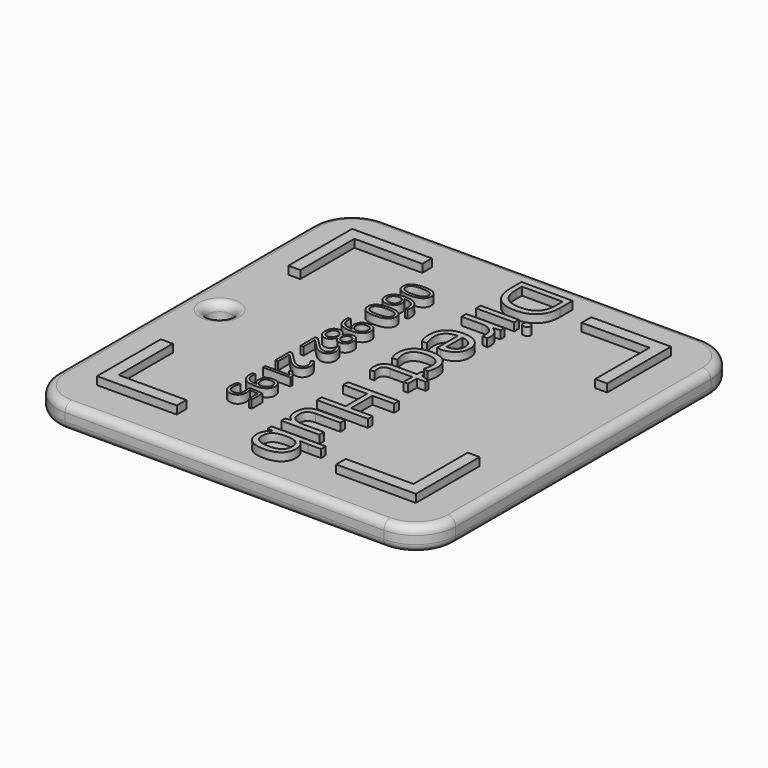
from build123d import *

# Parameters (mm, degrees)
F1_W          = 50
F1_H          = 50
F2_DEPTH      = 3
F4_D          = 3
F5_R          = 1
F6_R          = 1
F7_T1_DEPTH   = 3
F7_T4_ANGLE   = 90
F7_T6_ANGLE   = 90
F7_T8_ANGLE   = 90
F7_T10_ANGLE  = 90
F7_T12_ANGLE  = 90
F7_T14_ANGLE  = 90
F7_T16_ANGLE  = 90
F7_T18_ANGLE  = 90
F8_TEXT_SIZE  = 8.9550794579
F9_DEPTH      = 1
F10_TEXT_SIZE = 4.8044441108
F11_DEPTH     = 1
F13_DEPTH     = 1
F14_DEPTH     = 1


# Not quite as in the source:
# - a fillet or chamfer that OpenCascade refuses, or shapes differently, is made with other operations: its cross-section is extruded or revolved along the edge and cut away or added
# - Text() gives the source's letters only with a copy of the font that has no kerning and outlines rounded to 1/6400 em; it was checked with that copy


with BuildPart() as f2:
    # F1 (on face) → F2 (new body)
    with BuildSketch(Plane.XY):
        Rectangle(F1_W, F1_H)
    extrude(amount=F2_DEPTH)

    # F4 (through all)
    with Locations(Plane.XY.offset(3)):
        with Locations((-20.6191185862, 0)):
            Hole(F4_D / 2)

    # F5
    f5_edges = [f2.edges().sort_by_distance(p)[0] for p in [
        (-25, 0, 3),
        (0, 25, 3),
        (0, -25, 3),
        (25, 0, 3),
        (-22.119119, 0, 3),
    ]]
    fillet(f5_edges, radius=F5_R)

    # F6
    f6_edges = [f2.edges().sort_by_distance(p)[0] for p in [
        (-25, 0, 0),
        (0, 25, 0),
        (0, -25, 0),
        (25, 0, 0),
        (-22.119119, 0, 0),
    ]]
    fillet(f6_edges, radius=F6_R)

    # F7: fillet of radius 5 on 4 edges, made by hand

    # F7_s2 → F7_t1 (cut)
    with BuildSketch(Plane.XY):
        with BuildLine():
            ThreePointArc((-25, 20), (-23.5355339059, 23.5355339059), (-20, 25))
            Line((-20, 25), (-25, 25))
            Line((-25, 25), (-25, 20))
        make_face()
        with BuildLine():
            ThreePointArc((-25, -20), (-23.5355339059, -23.5355339059), (-20, -25))
            Line((-20, -25), (-25, -25))
            Line((-25, -25), (-25, -20))
        make_face()
        with BuildLine():
            ThreePointArc((20, 25), (23.5355339059, 23.5355339059), (25, 20))
            Line((25, 20), (25, 25))
            Line((25, 25), (20, 25))
        make_face()
        with BuildLine():
            ThreePointArc((20, -25), (23.5355339059, -23.5355339059), (25, -20))
            Line((25, -20), (25, -25))
            Line((25, -25), (20, -25))
        make_face()
    extrude(amount=F7_T1_DEPTH, mode=Mode.SUBTRACT)

    # F7_s3 → F7_t4 (revolve, cut)
    with BuildSketch(Plane.XZ.offset(20)):
        with BuildLine():
            ThreePointArc((24, 0), (24.7071067812, 0.2928932188), (25, 1))
            Line((25, 1), (25, 0))
            Line((25, 0), (24, 0))
        make_face()
    revolve(axis=Axis((20, -20, 0), (0, 0, -1)), revolution_arc=F7_T4_ANGLE, mode=Mode.SUBTRACT)

    # F7_s5 → F7_t6 (revolve, cut)
    with BuildSketch(Plane.YZ.offset(20)):
        with BuildLine():
            ThreePointArc((-24, 3), (-24.7071067812, 2.7071067812), (-25, 2))
            Line((-25, 2), (-25, 3))
            Line((-25, 3), (-24, 3))
        make_face()
    revolve(axis=Axis((20, -20, 3), (0, 0, 1)), revolution_arc=F7_T6_ANGLE, mode=Mode.SUBTRACT)

    # F7_s7 → F7_t8 (revolve, cut)
    with BuildSketch(Plane.YZ.offset(20)):
        with BuildLine():
            ThreePointArc((24, 0), (24.7071067812, 0.2928932188), (25, 1))
            Line((25, 1), (25, 0))
            Line((25, 0), (24, 0))
        make_face()
    revolve(axis=Axis((20, 20, 0), (0, 0, -1)), revolution_arc=F7_T8_ANGLE, mode=Mode.SUBTRACT)

    # F7_s9 → F7_t10 (revolve, cut)
    with BuildSketch(Plane.XZ.offset(-20)):
        with BuildLine():
            ThreePointArc((24, 3), (24.7071067812, 2.7071067812), (25, 2))
            Line((25, 2), (25, 3))
            Line((25, 3), (24, 3))
        make_face()
    revolve(axis=Axis((20, 20, 3), (0, 0, 1)), revolution_arc=F7_T10_ANGLE, mode=Mode.SUBTRACT)

    # F7_s11 → F7_t12 (revolve, cut)
    with BuildSketch(Plane.YZ.offset(-20)):
        with BuildLine():
            ThreePointArc((-24, 0), (-24.7071067812, 0.2928932188), (-25, 1))
            Line((-25, 1), (-25, 0))
            Line((-25, 0), (-24, 0))
        make_face()
    revolve(axis=Axis((-20, -20, 0), (0, 0, -1)), revolution_arc=F7_T12_ANGLE, mode=Mode.SUBTRACT)

    # F7_s13 → F7_t14 (revolve, cut)
    with BuildSketch(Plane.XZ.offset(20)):
        with BuildLine():
            ThreePointArc((-24, 3), (-24.7071067812, 2.7071067812), (-25, 2))
            Line((-25, 2), (-25, 3))
            Line((-25, 3), (-24, 3))
        make_face()
    revolve(axis=Axis((-20, -20, 3), (0, 0, 1)), revolution_arc=F7_T14_ANGLE, mode=Mode.SUBTRACT)

    # F7_s15 → F7_t16 (revolve, cut)
    with BuildSketch(Plane.XZ.offset(-20)):
        with BuildLine():
            ThreePointArc((-24, 0), (-24.7071067812, 0.2928932188), (-25, 1))
            Line((-25, 1), (-25, 0))
            Line((-25, 0), (-24, 0))
        make_face()
    revolve(axis=Axis((-20, 20, 0), (0, 0, -1)), revolution_arc=F7_T16_ANGLE, mode=Mode.SUBTRACT)

    # F7_s17 → F7_t18 (revolve, cut)
    with BuildSketch(Plane.YZ.offset(-20)):
        with BuildLine():
            ThreePointArc((24, 3), (24.7071067812, 2.7071067812), (25, 2))
            Line((25, 2), (25, 3))
            Line((25, 3), (24, 3))
        make_face()
    revolve(axis=Axis((-20, 20, 3), (0, 0, 1)), revolution_arc=F7_T18_ANGLE, mode=Mode.SUBTRACT)

    # F8 (on face) → F9 (join)
    with BuildSketch(Plane.XY.offset(3)):
        with Locations(Location((0, 22.4499644316), (0, 0, -90))):
            Text('Direct Hub', F8_TEXT_SIZE, font='Open Sans', text_align=(TextAlign.LEFT, TextAlign.BOTTOM))
    extrude(amount=F9_DEPTH)

    # F10 (on face) → F11 (join)
    with BuildSketch(Plane.XY.offset(3)):
        with Locations(Location((-8.4686320769, 15), (0, 0, -90))):
            Text('060 982 2195', F10_TEXT_SIZE, font='Open Sans', text_align=(TextAlign.LEFT, TextAlign.BOTTOM))
    extrude(amount=F11_DEPTH)

    # F12 (on face) → F13 (join)
    with BuildSketch(Plane.XY.offset(3)):
        Polygon((20, 10), (20, 20), (9.9999990551, 20), (9.9999990551, 18.5), (18.5, 18.510559866), (18.5, 10), align=None)
    extrude(amount=F13_DEPTH)

    # F12 (on face) → F14 (join)
    with BuildSketch(Plane.XY.offset(3)):
        Polygon((20, 10), (20, 20), (9.9999990551, 20), (9.9999990551, 18.5), (18.5, 18.510559866), (18.5, 10), align=None)
        Polygon((10, -20), (20, -20), (20, -10), (18.5, -10), (18.5, -18.51056), (10, -18.5), align=None)
        Polygon((-10, 20), (-20, 20), (-20, 10), (-18.5, 10), (-18.51, 18.5), (-10, 18.5), align=None)
        Polygon((-20, -10), (-20, -20), (-10, -20), (-10, -18.5), (-18.5, -18.5), (-18.5, -10), align=None)
    extrude(amount=F14_DEPTH)


solid = f2.part
